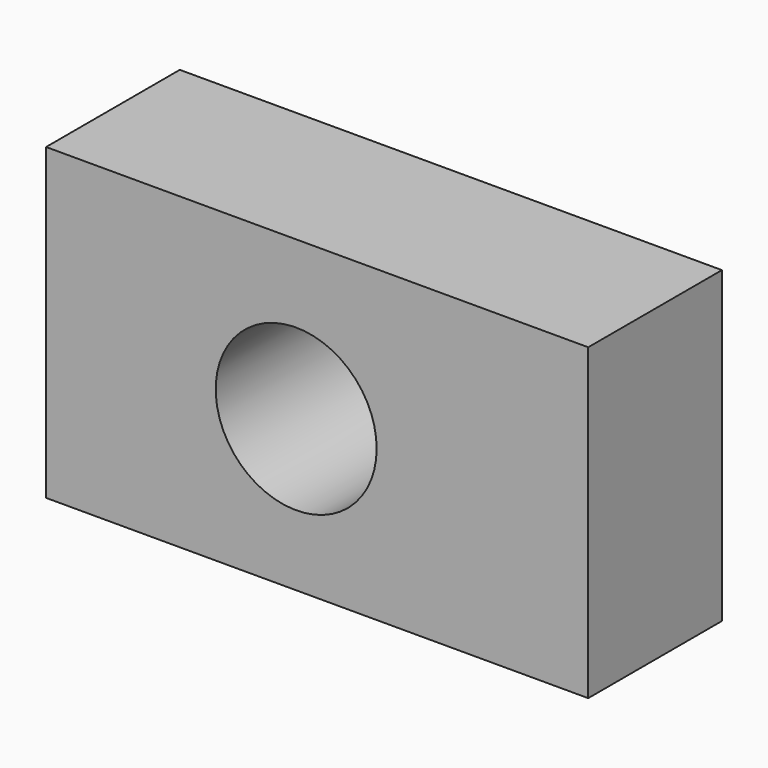
from build123d import *

# Parameters (mm, degrees)
F0_W     = 127.7268081903
F0_H     = 72.7801807225
F0_R     = 18.9582782215
F2_DEPTH = 39.37


# Not quite as in the source:
# - the program builds the solid bodies; features that only make, move or delete a surface that nothing else refers to are left out


with BuildPart() as f2:
    # F0 (on Front) → F2 (new body)
    with BuildSketch(Plane.XZ):
        with Locations((4.9403756857, 0.8434783667)):
            Rectangle(F0_W, F0_H)
        Circle(F0_R, mode=Mode.SUBTRACT)
    extrude(amount=F2_DEPTH)


solid = f2.part
